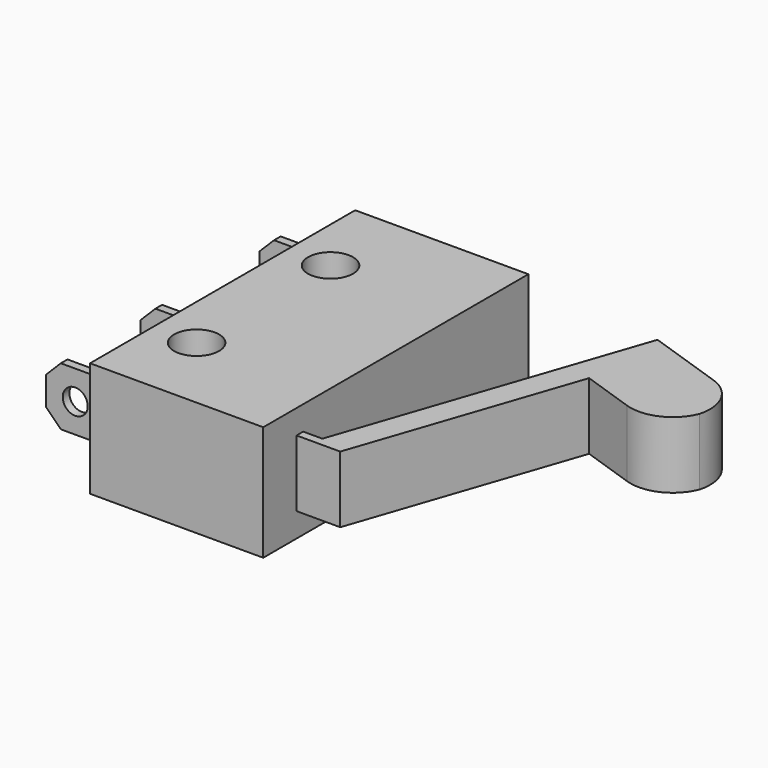
from build123d import *

# Parameters (mm, degrees)
F0_W         = 10.4
F0_H         = 19.9
F1_DEPTH     = 6.9
F2_R         = 1.35
F3_DEPTH     = 6.9
F4_W         = 0.5
F4_H         = 1.746198668
F5_DEPTH     = 4
F7_DEPTH     = 16.5
F8_W         = 0.5
F8_H         = 2
F9_DEPTH     = 1.15
F11_DEPTH    = 4
F12_W        = 1.55500961
F12_H        = 4
F13_DEPTH    = 18.65
F14_W        = 4.8
F14_H        = 4
F15_DEPTH    = 5.85
F16_T1_DEPTH = 16.7


# Not quite as in the source:
# - a fillet or chamfer that OpenCascade refuses, or shapes differently, is made with other operations: its cross-section is extruded or revolved along the edge and cut away or added


with BuildPart() as f1:
    # F0 (on Top) → F1 (new body)
    with BuildSketch(Plane.XY):
        Rectangle(F0_W, F0_H)
    extrude(amount=F1_DEPTH)

    # F2 (on face) → F3 (cut, through all)
    with BuildSketch(Plane.XY.offset(6.9)):
        with Locations((-2.6, 4.85)):
            Circle(F2_R)
        with Locations((-2.6, -5.2)):
            Circle(F2_R)
    extrude(amount=-F3_DEPTH, mode=Mode.SUBTRACT)

    # F4 (on face) → F5 (join)
    with BuildSketch(Plane(origin=(-5.2, 0, 0), x_dir=(0, -1, 0), z_dir=(-1, 0, 0))):
        with Locations((-8, 2.576900666)):
            Rectangle(F4_W, F4_H)
        with Locations((8, 4.323099334)):
            Rectangle(F4_W, F4_H)
        with Locations((8, 2.576900666)):
            Rectangle(F4_W, F4_H)
        with Locations((0.9, 4.323099334)):
            Rectangle(F4_W, F4_H)
        with Locations((0.9, 2.576900666)):
            Rectangle(F4_W, F4_H)
        with Locations((-8, 4.323099334)):
            Rectangle(F4_W, F4_H)
    extrude(amount=F5_DEPTH)

    # F6 (on face) → F7 (cut, through all)
    with BuildSketch(Plane(origin=(0, 8.25, 0), x_dir=(-1, 0, 0), z_dir=(0, 1, 0))):
        with BuildLine():
            Line((6.7, 3.45), (8.2, 3.45))
            ThreePointArc((8.2, 3.45), (7.45, 4.2), (6.7, 3.45))
        make_face()
        with BuildLine():
            ThreePointArc((6.7, 3.45), (7.45, 2.7), (8.2, 3.45))
            Line((8.2, 3.45), (6.7, 3.45))
        make_face()
        Polygon((9.2, 5.196198668), (8.3137443289, 5.196198668), (9.2, 4.3099429969), align=None)
        Polygon((9.2, 1.703801332), (9.2, 2.5900570031), (8.3137443289, 1.703801332), align=None)
    extrude(amount=-F7_DEPTH, mode=Mode.SUBTRACT)

    # F8 (on face) → F9 (join)
    with BuildSketch(Plane.YZ.offset(5.2)):
        with Locations((-7.2, 2.45)):
            Rectangle(F8_W, F8_H)
        with Locations((-7.2, 4.45)):
            Rectangle(F8_W, F8_H)
    extrude(amount=F9_DEPTH)

    # F10 (on face) → F11 (join, through all)
    with BuildSketch(Plane(origin=(0, 0, 1.45), x_dir=(1, 0, 0), z_dir=(0, 0, -1))):
        Polygon((6.35, 7.45), (6.35, 6.95), (7.8224316239, 7.45), align=None)
    extrude(amount=-F11_DEPTH)

    # F12 (on face) → F13 (join)
    with BuildSketch(Plane(origin=(-1.4595201755, -4.2980873242, 0), x_dir=(-0.946895514, 0.3215414212, 0), z_dir=(0.3215414212, 0.946895514, 0))):
        with Locations((-9.0250041964, 3.45)):
            Rectangle(F12_W, F12_H)
    extrude(amount=F13_DEPTH)

    # F14 (on face) → F15 (join)
    with BuildSketch(Plane(origin=(9.2819517994, -3.1519126758, 0), x_dir=(0.3215414212, 0.946895514, 0), z_dir=(0.946895514, -0.3215414212, 0))):
        with Locations((11.7108642024, 3.45)):
            Rectangle(F14_W, F14_H)
    extrude(amount=F15_DEPTH)

    # F16: fillet of radius 2.54 on 2 edges, made by hand

    # F16_s2 → F16_t1 (cut)
    with BuildSketch(Plane.XY.offset(-4.9)):
        with BuildLine():
            ThreePointArc((16.953403281, 9.145299232), (18.4148657814, 7.8633526103), (18.5418026766, 5.9234694165))
            Line((18.5418026766, 5.9234694165), (19.3585178865, 8.3285840221))
            Line((19.3585178865, 8.3285840221), (16.953403281, 9.145299232))
        make_face()
        with BuildLine():
            ThreePointArc((18.6318342746, 6.1886001604), (17.3498876529, 4.72713766), (15.4100044591, 4.6002007647))
            Line((15.4100044591, 4.6002007647), (17.8151190647, 3.7834855549))
            Line((17.8151190647, 3.7834855549), (18.6318342746, 6.1886001604))
        make_face()
    extrude(amount=F16_T1_DEPTH, mode=Mode.SUBTRACT)


solid = f1.part
